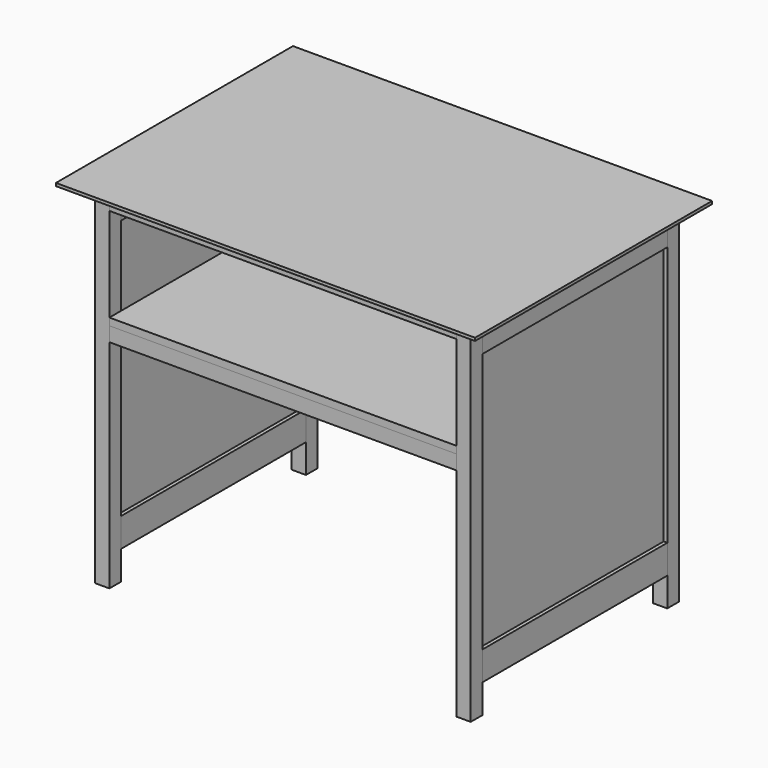
from build123d import *

# Parameters (mm, degrees)
F0_W      = 25.4
F0_H      = 25.4
F1_DEPTH  = 609.6
F2_W      = 25.4
F2_H      = 50.8
F3_DEPTH  = 406.4
F4_W      = 12.7
F4_H      = 457.2
F5_DEPTH  = 406.4
F6_W      = 25.4
F6_H      = 25.4
F7_DEPTH  = 609.6
F8_W      = 609.6
F8_H      = 12.7
F9_DEPTH  = 457.2
F10_W     = 736.6
F10_H     = 520.7
F10_W_2   = 25.4
F10_H_2   = 406.4
F11_DEPTH = 12.7
F12_SIZE2 = 19.05
F12_SIZE  = 7.62


with BuildPart() as f1:
    # F0 (on Top) → F1 (new body)
    with BuildSketch(Plane.XY):
        with Locations((-317.5, 215.9)):
            Rectangle(F0_W, F0_H)
    extrude(amount=F1_DEPTH)


with BuildPart() as f1b:
    # F0 (on Top) → F1, piece 2 (new body)
    with BuildSketch(Plane.XY):
        with Locations((317.5, 215.9)):
            Rectangle(F0_W, F0_H)
    extrude(amount=F1_DEPTH)


with BuildPart() as f1c:
    # F0 (on Top) → F1, piece 3 (new body)
    with BuildSketch(Plane.XY):
        with Locations((317.5, -215.9)):
            Rectangle(F0_W, F0_H)
    extrude(amount=F1_DEPTH)


with BuildPart() as f1d:
    # F0 (on Top) → F1, piece 4 (new body)
    with BuildSketch(Plane.XY):
        with Locations((-317.5, -215.9)):
            Rectangle(F0_W, F0_H)
    extrude(amount=F1_DEPTH)


with BuildPart() as f3:
    # F2 (on face) → F3 (new body, through all)
    with BuildSketch(Plane.XZ.offset(-203.2)):
        with Locations((-317.5, 584.2)):
            Rectangle(F2_W, F2_H)
    extrude(amount=F3_DEPTH)


with BuildPart() as f3b:
    # F2 (on face) → F3, piece 2 (new body, through all)
    with BuildSketch(Plane.XZ.offset(-203.2)):
        with Locations((317.5, 584.2)):
            Rectangle(F2_W, F2_H)
    extrude(amount=F3_DEPTH)


with BuildPart() as f3c:
    # F2 (on face) → F3, piece 3 (new body, through all)
    with BuildSketch(Plane.XZ.offset(-203.2)):
        with Locations((317.5, 76.2)):
            Rectangle(F2_W, F2_H)
    extrude(amount=F3_DEPTH)


with BuildPart() as f3d:
    # F2 (on face) → F3, piece 4 (new body, through all)
    with BuildSketch(Plane.XZ.offset(-203.2)):
        with Locations((-317.5, 76.2)):
            Rectangle(F2_W, F2_H)
    extrude(amount=F3_DEPTH)


with BuildPart() as f5:
    # F4 (on face) → F5 (new body, through all)
    with BuildSketch(Plane.XZ.offset(-203.2)):
        with Locations((317.5, 330.2)):
            Rectangle(F4_W, F4_H)
    extrude(amount=F5_DEPTH)


with BuildPart() as f5b:
    # F4 (on face) → F5, piece 2 (new body, through all)
    with BuildSketch(Plane.XZ.offset(-203.2)):
        with Locations((-317.5, 330.2)):
            Rectangle(F4_W, F4_H)
    extrude(amount=F5_DEPTH)


with BuildPart() as f7:
    # F6 (on face) → F7 (new body, through all)
    with BuildSketch(Plane(origin=(304.8, 0, 0), x_dir=(0, -1, 0), z_dir=(-1, 0, 0))):
        with Locations((-215.9, 596.9)):
            Rectangle(F6_W, F6_H)
    extrude(amount=F7_DEPTH)


with BuildPart() as f7b:
    # F6 (on face) → F7, piece 2 (new body, through all)
    with BuildSketch(Plane(origin=(304.8, 0, 0), x_dir=(0, -1, 0), z_dir=(-1, 0, 0))):
        with Locations((-215.9, 393.7)):
            Rectangle(F6_W, F6_H)
    extrude(amount=F7_DEPTH)


with BuildPart() as f7c:
    # F6 (on face) → F7, piece 3 (new body, through all)
    with BuildSketch(Plane(origin=(304.8, 0, 0), x_dir=(0, -1, 0), z_dir=(-1, 0, 0))):
        with Locations((215.9, 393.7)):
            Rectangle(F6_W, F6_H)
    extrude(amount=F7_DEPTH)


with BuildPart() as f7d:
    # F6 (on face) → F7, piece 4 (new body, through all)
    with BuildSketch(Plane(origin=(304.8, 0, 0), x_dir=(0, -1, 0), z_dir=(-1, 0, 0))):
        with Locations((215.9, 596.9)):
            Rectangle(F6_W, F6_H)
    extrude(amount=F7_DEPTH)


with BuildPart() as f9:
    # F8 (on face) → F9 (new body, through all)
    with BuildSketch(Plane.XZ.offset(228.6)):
        with Locations((0, 412.75)):
            Rectangle(F8_W, F8_H)
    extrude(amount=-F9_DEPTH)


with BuildPart() as f11:
    # F10 (on face) → F11 (new body)
    with BuildSketch(Plane.XY.offset(609.6)):
        with Locations((0, -6.35)):
            Rectangle(F10_W, F10_H)
        with Locations((-317.5, 0)):
            Rectangle(F10_W_2, F10_H_2, mode=Mode.SUBTRACT)
        with Locations((-317.5, 0)):
            Rectangle(F10_W_2, F10_H_2)
    extrude(amount=F11_DEPTH)

    # F12
    f12_edges = [f11.edges().sort_by_distance(p)[0] for p in [
        (0, -266.7, 609.6),
        (-368.3, -6.35, 609.6),
        (368.3, -6.35, 609.6),
        (0, 254, 609.6),
    ]]
    chamfer(f12_edges, length=F12_SIZE, length2=F12_SIZE2)


solid = Compound([f1.part, f1b.part, f1c.part, f1d.part, f3.part, f3b.part, f3c.part, f3d.part, f5.part, f5b.part, f7.part, f7b.part, f7c.part, f7d.part, f9.part, f11.part])
